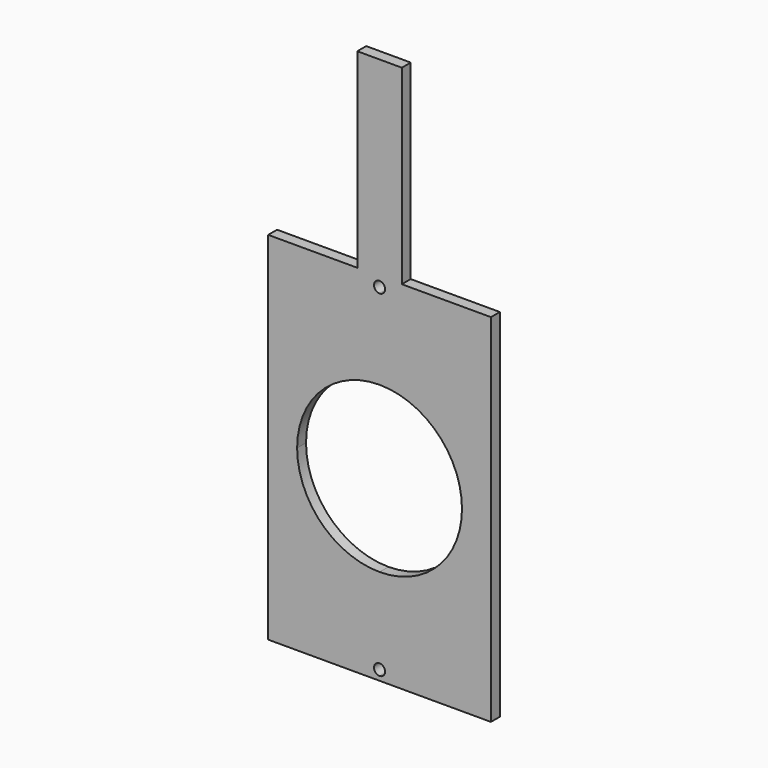
from build123d import *

# Parameters (mm, degrees)
F1_DEPTH = 3.175


# Not quite as in the source:
# - a feature names something its author has since deleted; it is built from what else it names


with BuildPart() as f1:
    # F0 (on Front) → F1 (new body)
    with BuildSketch(Plane.XZ):
        with BuildLine():
            Line((-94.8762850642, 108.0007998444), (-120.2762850642, 108.0007998444))
            Line((-120.2762850642, 108.0007998444), (-120.2762850642, 57.2007998444))
            Line((-120.2762850642, 57.2007998444), (-112.0251095462, 57.2007998444))
            ThreePointArc((-112.0251095462, 57.2007998444), (-105.1424632053, 73.8169779855), (-88.5262850642, 80.6996243264))
            Line((-88.5262850642, 80.6996243264), (-88.5262850642, 103.6132998444))
            ThreePointArc((-88.5262850642, 103.6132998444), (-90.1137850642, 105.2007998444), (-88.5262850642, 106.7882998444))
            Line((-88.5262850642, 106.7882998444), (-88.5262850642, 108.0007998444))
            Line((-88.5262850642, 108.0007998444), (-94.8762850642, 108.0007998444))
        make_face()
        with BuildLine():
            Line((-82.1762850642, 108.0007998444), (-88.5262850642, 108.0007998444))
            Line((-88.5262850642, 108.0007998444), (-88.5262850642, 106.7882998444))
            ThreePointArc((-88.5262850642, 106.7882998444), (-87.4037530491, 106.3233318595), (-86.9387850642, 105.2007998444))
            ThreePointArc((-86.9387850642, 105.2007998444), (-87.4037530491, 104.0782678293), (-88.5262850642, 103.6132998444))
            Line((-88.5262850642, 103.6132998444), (-88.5262850642, 80.6996243264))
            ThreePointArc((-88.5262850642, 80.6996243264), (-71.9101069231, 73.8169779855), (-65.0274605822, 57.2007998444))
            ThreePointArc((-65.0274605822, 57.2007998444), (-71.9101069231, 40.5846217033), (-88.5262850642, 33.7019753624))
            Line((-88.5262850642, 33.7019753624), (-88.5262850642, 10.7882998444))
            ThreePointArc((-88.5262850642, 10.7882998444), (-87.4037530491, 10.3233318595), (-86.9387850642, 9.2007998444))
            ThreePointArc((-86.9387850642, 9.2007998444), (-87.4037530491, 8.0782678293), (-88.5262850642, 7.6132998444))
            Line((-88.5262850642, 7.6132998444), (-88.5262850642, 6.4007998444))
            Line((-88.5262850642, 6.4007998444), (-56.7762850642, 6.4007998444))
            Line((-56.7762850642, 6.4007998444), (-56.7762850642, 108.0007998444))
            Line((-56.7762850642, 108.0007998444), (-82.1762850642, 108.0007998444))
        make_face()
        with BuildLine():
            Line((-112.0251095462, 57.2007998444), (-120.2762850642, 57.2007998444))
            Line((-120.2762850642, 57.2007998444), (-120.2762850642, 6.4007998444))
            Line((-120.2762850642, 6.4007998444), (-88.5262850642, 6.4007998444))
            Line((-88.5262850642, 6.4007998444), (-88.5262850642, 7.6132998444))
            ThreePointArc((-88.5262850642, 7.6132998444), (-90.1137850642, 9.2007998444), (-88.5262850642, 10.7882998444))
            Line((-88.5262850642, 10.7882998444), (-88.5262850642, 33.7019753624))
            ThreePointArc((-88.5262850642, 33.7019753624), (-105.1424632053, 40.5846217033), (-112.0251095462, 57.2007998444))
        make_face()
        Polygon((-94.8762850642, 162.3507998444), (-94.8762850642, 108.0007998444), (-88.5262850642, 108.0007998444), (-82.1762850642, 108.0007998444), (-82.1762850642, 162.3507998444), align=None)
    extrude(amount=F1_DEPTH)


solid = f1.part
